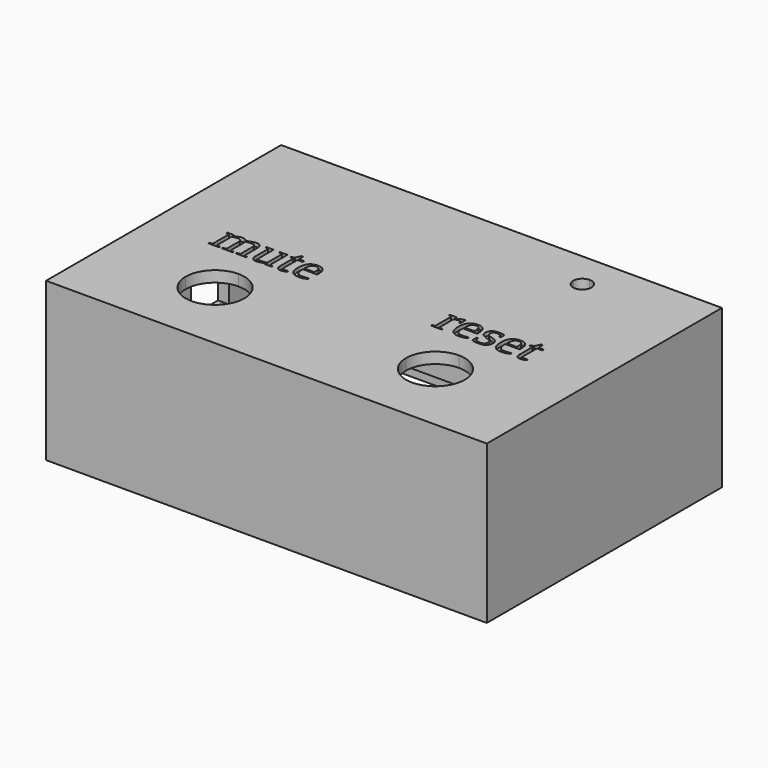
from build123d import *

# Parameters (mm, degrees)
F0_W         = 30
F0_H         = 10
F0_H_2       = 30
F1_DEPTH     = 3
F3_DEPTH     = 40
F4_W         = 117
F4_H         = 77
F4_W_2       = 114
F4_H_2       = 74
F5_DEPTH     = 3
F6_W         = 13
F6_H         = 11.5
F6_R         = 1.25
F7_DEPTH     = 25
F8_TEXT_SIZE = 13.8888888889
F9_DEPTH     = 1


# Not quite as in the source:
# - Text() gives the source's letters only with a copy of the font that has no kerning and outlines rounded to 1/6400 em; it was checked with that copy


with BuildPart() as f1:
    # F0 (on Top) → F1 (new body)
    with BuildSketch(Plane.XY):
        with Locations((-55.3229217822, 57.1930506412)):
            Rectangle(F0_W, F0_H)
        with Locations((-25.3229217822, 57.1930506412)):
            Rectangle(F0_W, F0_H)
        with Locations((-55.3229217822, 37.1930506412)):
            Rectangle(F0_W, F0_H_2)
        with BuildLine():
            Line((19.6770782178, 62.1930506412), (-10.3229217822, 62.1930506412))
            Line((-10.3229217822, 62.1930506412), (-10.3229217822, 52.1930506412))
            Line((-10.3229217822, 52.1930506412), (17.1770782178, 52.1930506412))
            ThreePointArc((17.1770782178, 52.1930506412), (17.9093112649, 53.9608175941), (19.6770782178, 54.6930506412))
            Line((19.6770782178, 54.6930506412), (19.6770782178, 62.1930506412))
        make_face()
        with BuildLine():
            Line((-40.3229217822, 22.1930506412), (-70.3229217822, 22.1930506412))
            Line((-70.3229217822, 22.1930506412), (-70.3229217822, 2.1930506412))
            Line((-70.3229217822, 2.1930506412), (-48.3229217822, 2.1930506412))
            ThreePointArc((-48.3229217822, 2.1930506412), (-45.9797760316, 7.8499048907), (-40.3229217822, 10.1930506412))
            Line((-40.3229217822, 10.1930506412), (-40.3229217822, 22.1930506412))
        make_face()
        with BuildLine():
            Line((49.6770782178, 62.1930506412), (19.6770782178, 62.1930506412))
            Line((19.6770782178, 62.1930506412), (19.6770782178, 54.6930506412))
            ThreePointArc((19.6770782178, 54.6930506412), (21.4448451708, 53.9608175941), (22.1770782178, 52.1930506412))
            Line((22.1770782178, 52.1930506412), (49.6770782178, 52.1930506412))
            Line((49.6770782178, 52.1930506412), (49.6770782178, 62.1930506412))
        make_face()
        with BuildLine():
            Line((-48.3229217822, 2.1930506412), (-70.3229217822, 2.1930506412))
            Line((-70.3229217822, 2.1930506412), (-70.3229217822, -17.8069493588))
            Line((-70.3229217822, -17.8069493588), (-40.3229217822, -17.8069493588))
            Line((-40.3229217822, -17.8069493588), (-40.3229217822, -5.8069493588))
            ThreePointArc((-40.3229217822, -5.8069493588), (-45.9797760316, -3.4638036083), (-48.3229217822, 2.1930506412))
        make_face()
        with BuildLine():
            Line((49.6770782178, 22.1930506412), (49.6770782178, 52.1930506412))
            Line((49.6770782178, 52.1930506412), (22.1770782178, 52.1930506412))
            ThreePointArc((22.1770782178, 52.1930506412), (21.4448451708, 50.4252836882), (19.6770782178, 49.6930506412))
            Line((19.6770782178, 49.6930506412), (19.6770782178, 22.1930506412))
            Line((19.6770782178, 22.1930506412), (49.6770782178, 22.1930506412))
        make_face()
        with BuildLine():
            Line((11.6770782178, 2.1930506412), (-10.3229217822, 2.1930506412))
            Line((-10.3229217822, 2.1930506412), (-10.3229217822, -17.8069493588))
            Line((-10.3229217822, -17.8069493588), (19.6770782178, -17.8069493588))
            Line((19.6770782178, -17.8069493588), (19.6770782178, -5.8069493588))
            ThreePointArc((19.6770782178, -5.8069493588), (14.0202239684, -3.4638036083), (11.6770782178, 2.1930506412))
        make_face()
        with BuildLine():
            Line((-10.3229217822, -17.8069493588), (-10.3229217822, 2.1930506412))
            Line((-10.3229217822, 2.1930506412), (-32.3229217822, 2.1930506412))
            ThreePointArc((-32.3229217822, 2.1930506412), (-34.6660675327, -3.4638036083), (-40.3229217822, -5.8069493588))
            Line((-40.3229217822, -5.8069493588), (-40.3229217822, -17.8069493588))
            Line((-40.3229217822, -17.8069493588), (-10.3229217822, -17.8069493588))
        make_face()
        with BuildLine():
            Line((49.6770782178, 22.1930506412), (19.6770782178, 22.1930506412))
            Line((19.6770782178, 22.1930506412), (19.6770782178, 10.1930506412))
            ThreePointArc((19.6770782178, 10.1930506412), (25.3339324673, 7.8499048907), (27.6770782178, 2.1930506412))
            Line((27.6770782178, 2.1930506412), (49.6770782178, 2.1930506412))
            Line((49.6770782178, 2.1930506412), (49.6770782178, 22.1930506412))
        make_face()
        with BuildLine():
            Line((49.6770782178, -17.8069493588), (49.6770782178, 2.1930506412))
            Line((49.6770782178, 2.1930506412), (27.6770782178, 2.1930506412))
            ThreePointArc((27.6770782178, 2.1930506412), (25.3339324673, -3.4638036083), (19.6770782178, -5.8069493588))
            Line((19.6770782178, -5.8069493588), (19.6770782178, -17.8069493588))
            Line((19.6770782178, -17.8069493588), (49.6770782178, -17.8069493588))
        make_face()
        with Locations((-25.3229217822, 37.1930506412)):
            Rectangle(F0_W, F0_H_2)
        with BuildLine():
            Line((17.1770782178, 52.1930506412), (-10.3229217822, 52.1930506412))
            Line((-10.3229217822, 52.1930506412), (-10.3229217822, 22.1930506412))
            Line((-10.3229217822, 22.1930506412), (19.6770782178, 22.1930506412))
            Line((19.6770782178, 22.1930506412), (19.6770782178, 49.6930506412))
            ThreePointArc((19.6770782178, 49.6930506412), (17.9093112649, 50.4252836882), (17.1770782178, 52.1930506412))
        make_face()
        with BuildLine():
            Line((19.6770782178, 22.1930506412), (-10.3229217822, 22.1930506412))
            Line((-10.3229217822, 22.1930506412), (-10.3229217822, 2.1930506412))
            Line((-10.3229217822, 2.1930506412), (11.6770782178, 2.1930506412))
            ThreePointArc((11.6770782178, 2.1930506412), (14.0202239684, 7.8499048907), (19.6770782178, 10.1930506412))
            Line((19.6770782178, 10.1930506412), (19.6770782178, 22.1930506412))
        make_face()
        with BuildLine():
            Line((-10.3229217822, 22.1930506412), (-40.3229217822, 22.1930506412))
            Line((-40.3229217822, 22.1930506412), (-40.3229217822, 10.1930506412))
            ThreePointArc((-40.3229217822, 10.1930506412), (-34.6660675327, 7.8499048907), (-32.3229217822, 2.1930506412))
            Line((-32.3229217822, 2.1930506412), (-10.3229217822, 2.1930506412))
            Line((-10.3229217822, 2.1930506412), (-10.3229217822, 22.1930506412))
        make_face()
    extrude(amount=F1_DEPTH)

    # F2 (on face) → F3 (join)
    with BuildSketch(Plane.XY):
        Polygon((-40.3229217822, -14.8069493588), (-67.3229217822, -14.8069493588), (-67.3229217822, 2.1930506412), (-70.3229217822, 2.1930506412), (-70.3229217822, -17.8069493588), (-40.3229217822, -17.8069493588), align=None)
        Polygon((46.6770782178, -14.8069493588), (-40.3229217822, -14.8069493588), (-40.3229217822, -17.8069493588), (49.6770782178, -17.8069493588), (49.6770782178, 62.1930506412), (-70.3229217822, 62.1930506412), (-70.3229217822, 2.1930506412), (-67.3229217822, 2.1930506412), (-67.3229217822, 59.1930506412), (46.6770782178, 59.1930506412), align=None)
    extrude(amount=-F3_DEPTH)

    # F4 (on face) → F5 (cut)
    with BuildSketch(Plane(origin=(0, 0, -40), x_dir=(1, 0, 0), z_dir=(0, 0, -1))):
        with Locations((-10.3229217822, -22.1930506412)):
            Rectangle(F4_W, F4_H)
        with Locations((-10.3229217822, -22.1930506412)):
            Rectangle(F4_W_2, F4_H_2, mode=Mode.SUBTRACT)
    extrude(amount=-F5_DEPTH, mode=Mode.SUBTRACT)

    # F6 (on face) → F7 (cut)
    with BuildSketch(Plane.YZ.offset(-67.3229217822)):
        with Locations((34.1930506412, -19.75)):
            Rectangle(F6_W, F6_H)
        with Locations((-5.8069493588, -9)):
            Circle(F6_R)
    extrude(amount=-F7_DEPTH, mode=Mode.SUBTRACT)

    # F8 (on face) → F9 (cut)
    with BuildSketch(Plane.XY.offset(3)):
        with Locations((-54.4016978238, 17.1930506412)):
            Text('mute', F8_TEXT_SIZE, font='Tinos', text_align=(TextAlign.LEFT, TextAlign.BOTTOM))
        with Locations((6.1733889817, 17.1930506412)):
            Text('reset', F8_TEXT_SIZE, font='Tinos', text_align=(TextAlign.LEFT, TextAlign.BOTTOM))
    extrude(amount=-F9_DEPTH, mode=Mode.SUBTRACT)


solid = f1.part
